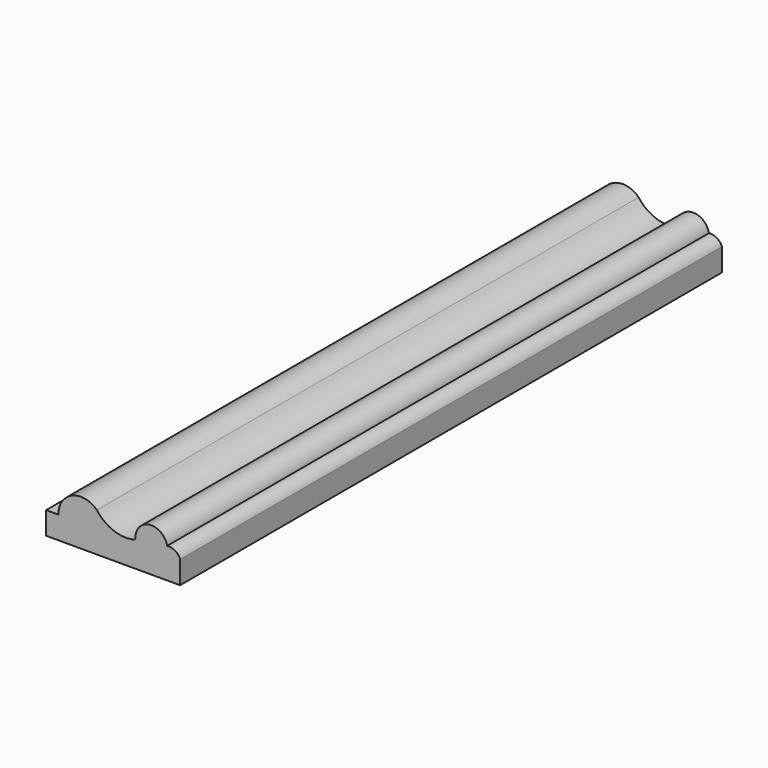
from build123d import *

# Parameters (mm, degrees)
F1_DEPTH = 152.4


# Not quite as in the source:
# - ends of sketch curves that miss each other by under 0.0002 mm in the source are joined


with BuildPart() as f1:
    # F0 (on Front) → F1 (new body)
    with BuildSketch(Plane.XZ):
        with BuildLine():
            Line((-15.08125, -0.0575056), (-15.08125, -5.1375056))
            Line((-15.08125, -5.1375056), (15.08125, -5.1375056))
            Line((15.08125, -5.1375056), (15.08125, 0.0021844))
            ThreePointArc((15.08125, 0.0021844), (13.9110698555, 1.3548551921), (12.1602591961, 1.7204961727))
            ThreePointArc((12.1602591961, 1.7204961727), (8.2596509367, 4.6235312638), (5.0188785469, 0.9986517001))
            ThreePointArc((5.0188785469, 0.9986517001), (4.9172605863, 0.6881685275), (4.6475872685, 0.5037694102))
            ThreePointArc((4.6475872685, 0.5037694102), (0.024076878, 0.8584026505), (-3.6593765677, 3.6752794438))
            ThreePointArc((-3.6593765677, 3.6752794438), (-9.2418941924, 4.7215006609), (-12.3111241543, -0.0575061109))
            Line((-12.3111241543, -0.0575061109), (-15.08125, -0.0575056))
        make_face()
    extrude(amount=F1_DEPTH)


solid = f1.part
